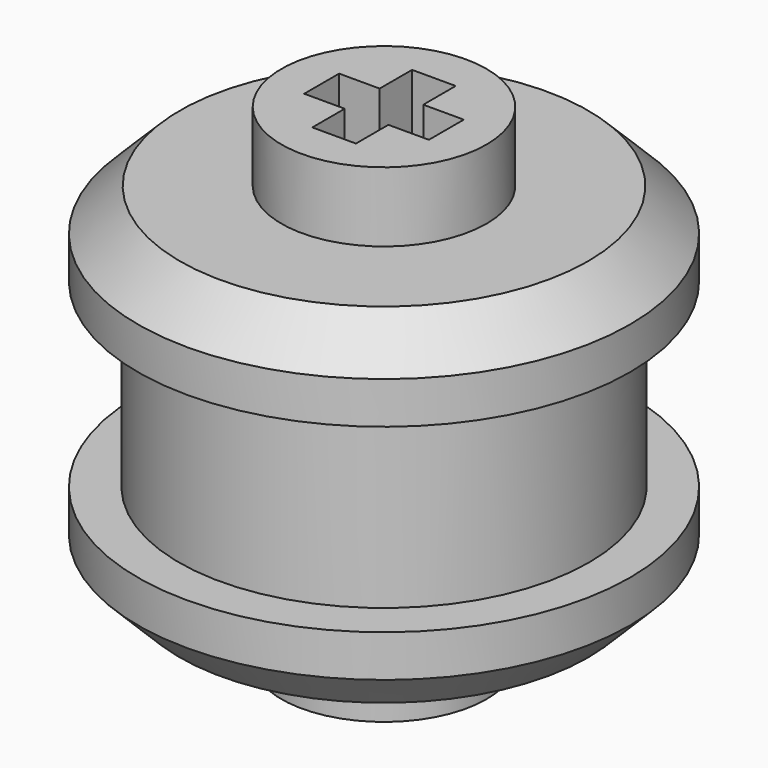
from build123d import *

# Parameters (mm, degrees)
F0_R      = 7.9375
F1_DEPTH  = 7
F2_R      = 9.525
F2_R_2    = 7.9375
F3_DEPTH  = 3.2512
F4_R      = 9.525
F4_R_2    = 7.9375
F5_DEPTH  = 3.2512
F6_SIZE   = 1.6256
F7_R      = 3.96875
F8_DEPTH  = 2.6975943
F9_R      = 3.96875
F10_DEPTH = 2.6975943


with BuildPart() as f1:
    # F0 (on Top) → F1 (new body)
    with BuildSketch(Plane.XY):
        Circle(F0_R)
        Polygon((0.84455, 0.84455), (2.413, 0.84455), (2.413, -0.84455), (0.84455, -0.84455), (0.84455, -2.413), (-0.84455, -2.413), (-0.84455, -0.84455), (-2.413, -0.84455), (-2.413, 0.84455), (-0.84455, 0.84455), (-0.84455, 2.413), (0.84455, 2.413), align=None, mode=Mode.SUBTRACT)
    extrude(amount=F1_DEPTH)

    # F2 (on face) → F3 (join)
    with BuildSketch(Plane.XY.offset(7)):
        Circle(F2_R)
        Circle(F2_R_2, mode=Mode.SUBTRACT)
        Circle(F2_R_2)
        Polygon((0.84455, 2.413), (0.84455, 0.84455), (2.413, 0.84455), (2.413, -0.84455), (0.84455, -0.84455), (0.84455, -2.413), (-0.84455, -2.413), (-0.84455, -0.84455), (-2.413, -0.84455), (-2.413, 0.84455), (-0.84455, 0.84455), (-0.84455, 2.413), align=None, mode=Mode.SUBTRACT)
    extrude(amount=F3_DEPTH)

    # F4 (on face) → F5 (join)
    with BuildSketch(Plane(origin=(0, 0, 0), x_dir=(1, 0, 0), z_dir=(0, 0, -1))):
        Circle(F4_R)
        Circle(F4_R_2, mode=Mode.SUBTRACT)
        Circle(F4_R_2)
        Polygon((2.413, 0.84455), (2.413, -0.84455), (0.84455, -0.84455), (0.84455, -2.413), (-0.84455, -2.413), (-0.84455, -0.84455), (-2.413, -0.84455), (-2.413, 0.84455), (-0.84455, 0.84455), (-0.84455, 2.413), (0.84455, 2.413), (0.84455, 0.84455), align=None, mode=Mode.SUBTRACT)
    extrude(amount=F5_DEPTH)

    # F6
    f6_edges = [f1.edges().sort_by_distance(p)[0] for p in [
        (-9.525, 0, 10.2512),
        (-9.525, 0, -3.2512),
    ]]
    chamfer(f6_edges, length=F6_SIZE)

    # F7 (on face) → F8 (join)
    with BuildSketch(Plane.XY.offset(10.2512)):
        Circle(F7_R)
        Polygon((-2.413, -0.84455), (-2.413, 0.84455), (-0.84455, 0.84455), (-0.84455, 2.413), (0.84455, 2.413), (0.84455, 0.84455), (2.413, 0.84455), (2.413, -0.84455), (0.84455, -0.84455), (0.84455, -2.413), (-0.84455, -2.413), (-0.84455, -0.84455), align=None, mode=Mode.SUBTRACT)
    extrude(amount=F8_DEPTH)

    # F9 (on face) → F10 (join)
    with BuildSketch(Plane(origin=(0, 0, -3.2512), x_dir=(1, 0, 0), z_dir=(0, 0, -1))):
        Circle(F9_R)
        Polygon((-0.84455, 2.413), (0.84455, 2.413), (0.84455, 0.84455), (2.413, 0.84455), (2.413, -0.84455), (0.84455, -0.84455), (0.84455, -2.413), (-0.84455, -2.413), (-0.84455, -0.84455), (-2.413, -0.84455), (-2.413, 0.84455), (-0.84455, 0.84455), align=None, mode=Mode.SUBTRACT)
    extrude(amount=F10_DEPTH)


solid = f1.part
